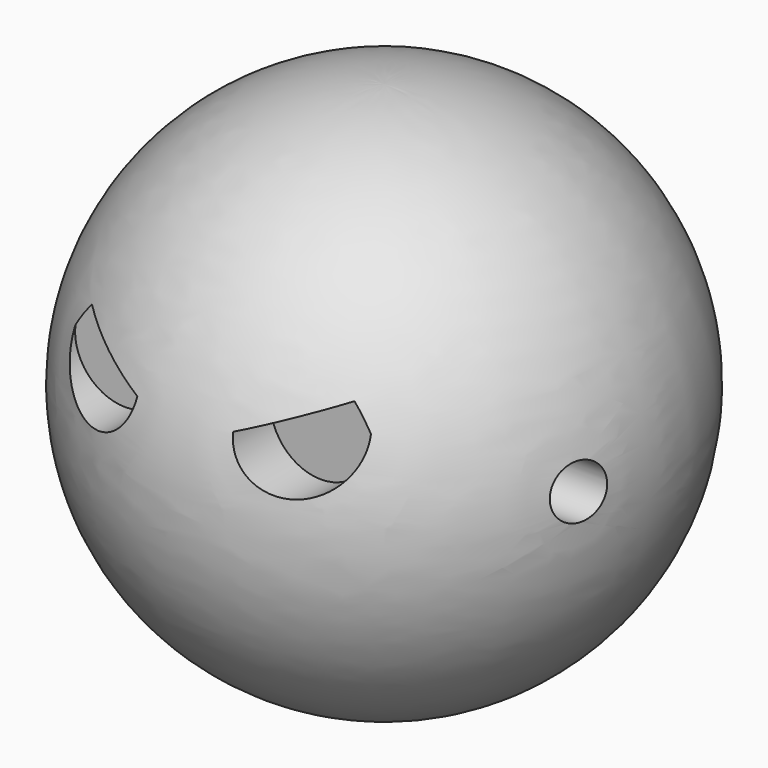
from build123d import *

# Parameters (mm, degrees)
F5_DEPTH  = 13.97
F6_R      = 1.5
F7_DEPTH  = 15.24
F8_W      = 36.1250601709
F8_H      = 9.7824148252
F9_DEPTH  = 76.2
F10_R     = 1.5
F11_DEPTH = 2.794


# Not quite as in the source:
# - ends of sketch curves that miss each other by under 0.0002 mm in the source are joined


with BuildPart() as f1:
    # F0 (on Front) → F1 (revolve)
    with BuildSketch(Plane.XZ):
        with BuildLine():
            Line((0, 30), (0, 0))
            ThreePointArc((0, 0), (15.0000006192, 15), (0, 30))
        make_face()
    revolve(axis=Axis((0, 0, 15), (0, 0, 1)))

    # F4 (on offset) → F5 (cut)
    with BuildSketch(Plane.XZ.offset(25.4)):
        with BuildLine():
            ThreePointArc((-7.7757835388, 21.3449876755), (-6.6607308484, 16.8981042804), (-2.7180244215, 19.2375872284))
            Line((-2.7180244215, 19.2375872284), (-7.7757835388, 21.3449876755))
        make_face()
        with BuildLine():
            Line((7.7757835388, 21.3449876755), (2.7180244215, 19.2375872284))
            ThreePointArc((2.7180244215, 19.2375872284), (6.6607308484, 16.8981042804), (7.7757835388, 21.3449876755))
        make_face()
    extrude(amount=-F5_DEPTH, mode=Mode.SUBTRACT)

    # F6 (on offset) → F7 (cut)
    with BuildSketch(Plane.YZ.offset(25.4)):
        with Locations((-4.0855947882, 15.938160941)):
            Circle(F6_R)
    extrude(amount=-F7_DEPTH, mode=Mode.SUBTRACT)

    # F8 (on offset) → F9 (cut)
    with BuildSketch(Plane.XZ.offset(25.4)):
        with Locations((1.2260917574, -4.0021650784)):
            Rectangle(F8_W, F8_H)
    extrude(amount=-F9_DEPTH, mode=Mode.SUBTRACT)

    # F10 (on face) → F11 (cut)
    with BuildSketch(Plane(origin=(0, 0, 0.8890423342), x_dir=(1, 0, 0), z_dir=(0, 0, -1))):
        Circle(F10_R)
    extrude(amount=-F11_DEPTH, mode=Mode.SUBTRACT)


solid = f1.part
